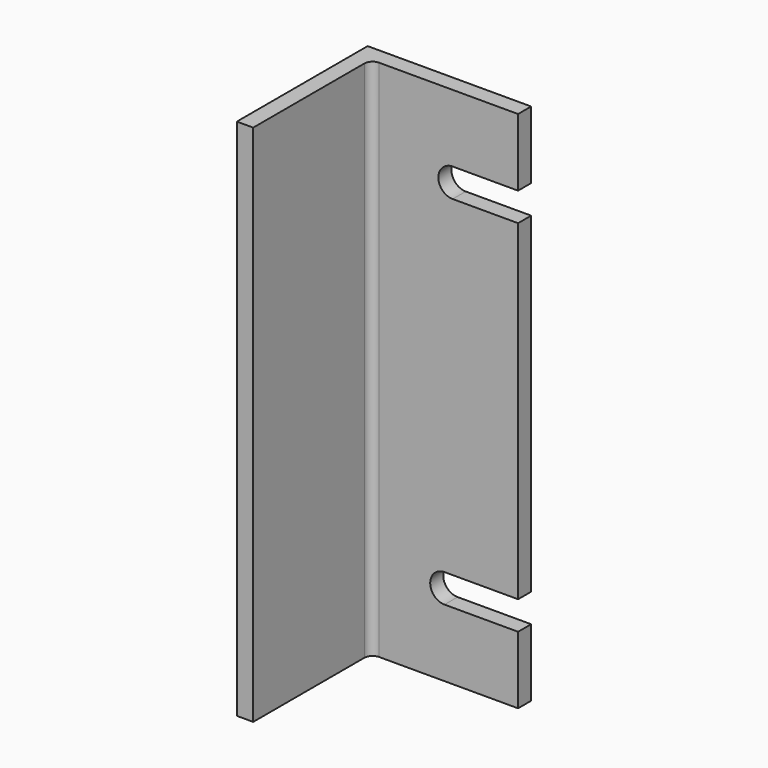
from build123d import *

# Parameters (mm, degrees)
F1_DEPTH = 203.2
F3_DEPTH = 25.4


# Not quite as in the source:
# - ends of sketch curves that miss each other by under 0.0002 mm in the source are joined


with BuildPart() as f1:
    # F0 (on Top) → F1 (new body)
    with BuildSketch(Plane.XY):
        with BuildLine():
            Line((0, -6.35), (0, -63.5))
            Line((0, -63.5), (6.35, -63.5))
            Line((6.35, -63.5), (6.35, -9.525))
            ThreePointArc((6.35, -9.525), (7.2799359697, -7.2799359697), (9.525, -6.35))
            Line((9.525, -6.35), (63.5, -6.35))
            Line((63.5, -6.35), (63.5, 0))
            Line((63.5, 0), (6.35, 0))
            Line((6.35, 0), (0, 0))
            Line((0, 0), (0, -6.35))
        make_face()
    extrude(amount=F1_DEPTH)

    # F2 (on face) → F3 (cut)
    with BuildSketch(Plane.XZ.offset(6.35)):
        with BuildLine():
            Line((38.1, 165.8788350046), (63.5, 165.8788350046))
            Line((63.5, 165.8788350046), (63.5, 176.9913350046))
            Line((63.5, 176.9913350046), (38.1, 176.9913350046))
            ThreePointArc((38.1, 176.9913350046), (32.54375, 171.4350850046), (38.1, 165.8788350046))
        make_face()
        with BuildLine():
            Line((34.925, 37.2913350046), (34.8918574917, 37.2913350046))
            ThreePointArc((34.8918574917, 37.2913350046), (29.3687747109, 31.7185139715), (34.925, 26.1788350046))
            Line((34.925, 26.1788350046), (63.5, 26.1788350046))
            Line((63.5, 26.1788350046), (63.5, 37.2913350046))
            Line((63.5, 37.2913350046), (34.925, 37.2913350046))
        make_face()
    extrude(amount=-F3_DEPTH, mode=Mode.SUBTRACT)


solid = f1.part
